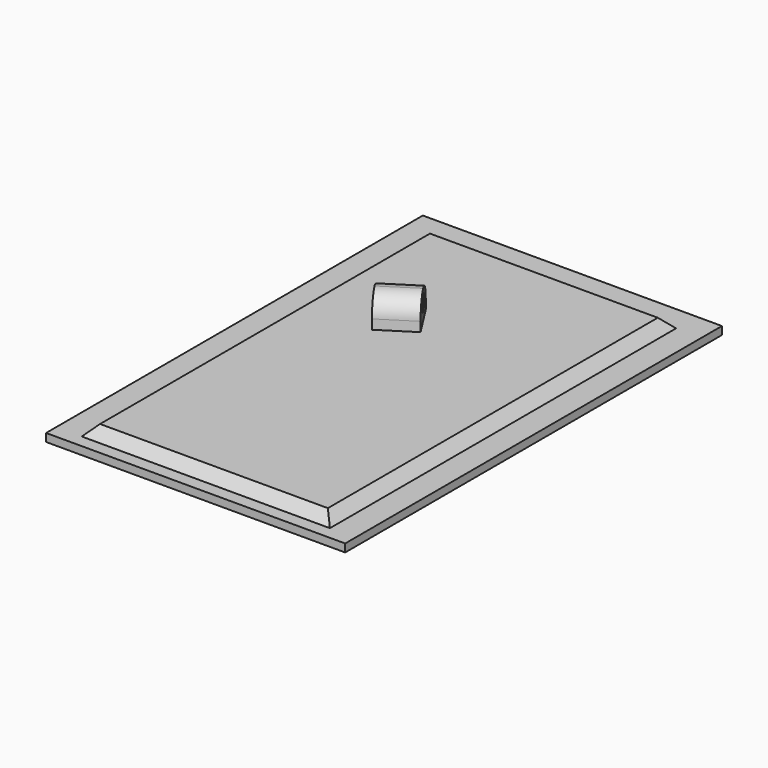
from build123d import *

# Parameters (mm, degrees)
F0_W     = 94
F0_H     = 148
F0_W_2   = 78
F0_H_2   = 136
F1_DEPTH = 2.5
F2_DEPTH = 3.2
F3_SIZE  = 3.19999
F6_DEPTH = 9
F7_R     = 5.99999
F8_R     = 2.5
F9_DEPTH = 12.1


# Not quite as in the source:
# - a fillet or chamfer is up to 0.001 mm smaller than in the source, because OpenCascade refuses the exact size


with BuildPart() as f1:
    # F0 (on Top) → F1 (new body)
    with BuildSketch(Plane.XY):
        Rectangle(F0_W, F0_H)
        with Locations((0, -2)):
            Rectangle(F0_W_2, F0_H_2, mode=Mode.SUBTRACT)
        with Locations((0, -2)):
            Rectangle(F0_W_2, F0_H_2)
    extrude(amount=-F1_DEPTH)

    # F0 (on Top) → F2 (join)
    with BuildSketch(Plane.XY):
        with Locations((0, -2)):
            Rectangle(F0_W_2, F0_H_2)
    extrude(amount=F2_DEPTH)

    # F3 (size 3.2 in the source; OpenCascade refuses exactly that, so slightly less here)
    f3_edges = [f1.edges().sort_by_distance(p)[0] for p in [
        (-39, -2, 3.2),
        (0, -70, 3.2),
        (39, -2, 3.2),
        (0, 66, 3.2),
    ]]
    chamfer(f3_edges, length=F3_SIZE)

    # F5 (on face) → F6 (join)
    with BuildSketch(Plane.XY.offset(3.2)):
        Polygon((-21.4385061716, 24.1024312943), (-19.825111455, 21.5732105668), (-14.9849273053, 13.9855483843), (-4.8680443952, 20.4391272506), (-11.3216232616, 30.5560101607), align=None)
    extrude(amount=F6_DEPTH)

    # F7 (radius 6 in the source; OpenCascade refuses exactly that, so slightly less here)
    f7_edges = [f1.edges().sort_by_distance(p)[0] for p in [
        (-9.926486, 17.212338, 12.2),
        (-16.380065, 27.329221, 12.2),
    ]]
    fillet(f7_edges, radius=F7_R)

    # F8 (on face) → F9 (cut)
    with BuildSketch(Plane(origin=(-4.3097861814, -2.749220809, 0), x_dir=(0.5377982389, -0.8430735758, 0), z_dir=(-0.8430735758, -0.5377982389, 0))):
        with Locations((-25.8497138006, 8.2)):
            Circle(F8_R)
    extrude(amount=-F9_DEPTH, mode=Mode.SUBTRACT)


solid = f1.part
